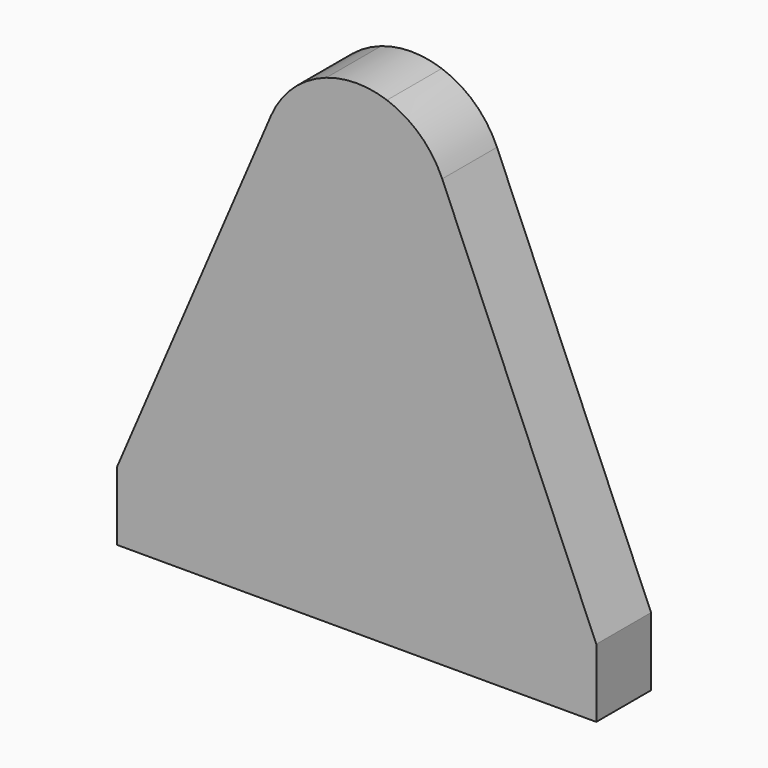
from build123d import *

# Parameters (mm, degrees)
F0_W     = 140
F0_H     = 20
F1_DEPTH = 20
F3_DEPTH = 5


with BuildPart() as f1:
    # F0 (on Front) → F1 (new body)
    with BuildSketch(Plane.XZ):
        with Locations((0, -60)):
            Rectangle(F0_W, F0_H)
        with BuildLine():
            Line((-70, -50), (70, -50))
            Line((70, -50), (25, 55))
            ThreePointArc((25, 55), (18.5187341548, 64.2068689629), (8.8640526043, 70))
            Line((8.8640526043, 70), (-8.8640526043, 70))
            ThreePointArc((-8.8640526043, 70), (-18.5187341548, 64.2068689629), (-25, 55))
            Line((-25, 55), (-70, -50))
        make_face()
        with BuildLine():
            Line((-8.8640526043, 70), (8.8640526043, 70))
            ThreePointArc((8.8640526043, 70), (0, 71.4849039495), (-8.8640526043, 70))
        make_face()
    extrude(amount=F1_DEPTH)

    # F2 (on face) → F3 (cut)
    with BuildSketch(Plane(origin=(0, 0, 0), x_dir=(-1, 0, 0), z_dir=(0, 1, 0))):
        with BuildLine():
            ThreePointArc((11, 51.4849039495), (7.7781745931, 59.2630785426), (0, 62.4849039495))
            ThreePointArc((0, 62.4849039495), (-7.7781745931, 43.7067293565), (11, 51.4849039495))
        make_face()
    extrude(amount=-F3_DEPTH, mode=Mode.SUBTRACT)


solid = f1.part
